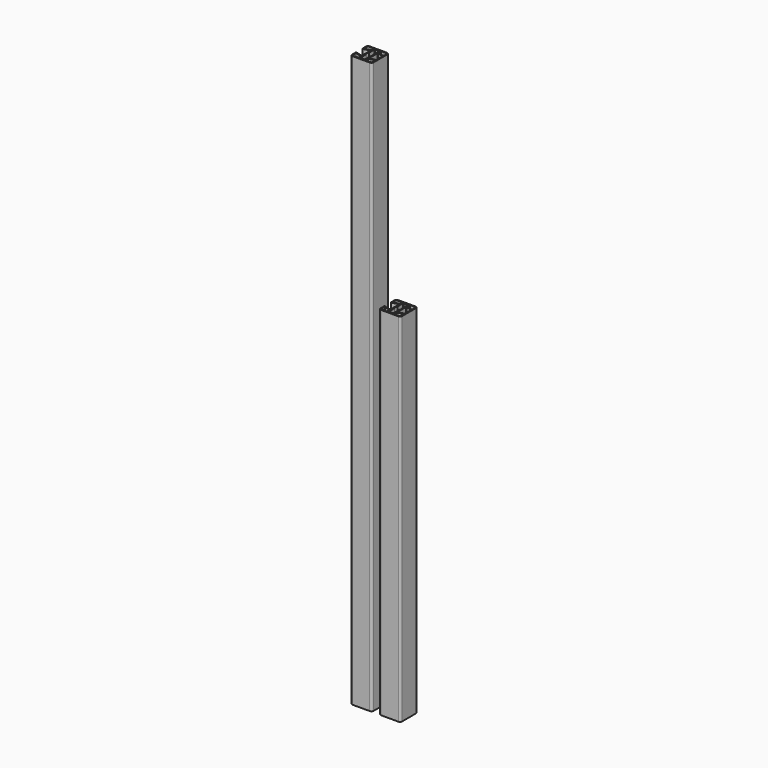
from build123d import *

# Parameters (mm, degrees)
F1_DEPTH = 1600
F2_DEPTH = 1000


# Not quite as in the source:
# - ends of sketch curves that miss each other by under 0.0002 mm in the source are joined


with BuildPart() as f1:
    # F0 (on Top) → F1 (new body)
    with BuildSketch(Plane.XY):
        with BuildLine():
            ThreePointArc((-11.2588189596, 15.2716838492), (-10.3912385359, 15.0991113133), (-10, 14.305758))
            Line((-10, 14.305758), (-10, -14.305758))
            ThreePointArc((-10, -14.305758), (-10.3912385359, -15.0991113133), (-11.2588189596, -15.2716838492))
            Line((-11.2588189596, -15.2716838492), (-28.426476, -10.671624))
            ThreePointArc((-28.426476, -10.671624), (-29.5109517857, -10.8873403242), (-30, -11.879032))
            Line((-30, -11.879032), (-30, -24))
            ThreePointArc((-30, -24), (-28.2426406871, -28.2426406871), (-24, -30))
            Line((-24, -30), (24, -30))
            ThreePointArc((24, -30), (28.2426406871, -28.2426406871), (30, -24))
            Line((30, -24), (30, 24))
            ThreePointArc((30, 24), (28.2426406871, 28.2426406871), (24, 30))
            Line((24, 30), (-24, 30))
            ThreePointArc((-24, 30), (-28.2426406871, 28.2426406871), (-30, 24))
            Line((-30, 24), (-30, 11.879032))
            ThreePointArc((-30, 11.879032), (-29.5109517857, 10.8873403242), (-28.4264761923, 10.6716247175))
            Line((-28.4264761923, 10.6716247175), (-11.2588189596, 15.2716838492))
        make_face()
        with BuildLine():
            Line((-11, -27.25), (-24, -27.25))
            ThreePointArc((-24, -27.25), (-26.2980970389, -26.2980970389), (-27.25, -24))
            Line((-27.25, -24), (-27.25, -15.137095))
            ThreePointArc((-27.25, -15.137095), (-26.8587614641, -14.3437416867), (-25.9911810404, -14.1711691508))
            Line((-25.9911810404, -14.1711691508), (-10.741181, -18.257395))
            ThreePointArc((-10.741181, -18.257395), (-10.2066466079, -18.6145586385), (-10, -19.22332))
            Line((-10, -19.22332), (-10, -26.25))
            ThreePointArc((-10, -26.25), (-10.2928932188, -26.9571067812), (-11, -27.25))
        make_face(mode=Mode.SUBTRACT)
        with BuildLine():
            Line((10.741181, -18.257395), (25.991181, -14.171169))
            ThreePointArc((25.991181, -14.171169), (26.8587614641, -14.3437416867), (27.25, -15.137095))
            Line((27.25, -15.137095), (27.25, -24))
            ThreePointArc((27.25, -24), (26.2980970389, -26.2980970389), (24, -27.25))
            Line((24, -27.25), (11, -27.25))
            ThreePointArc((11, -27.25), (10.2928932188, -26.9571067812), (10, -26.25))
            Line((10, -26.25), (10, -19.22332))
            ThreePointArc((10, -19.22332), (10.2066466079, -18.6145586385), (10.741181, -18.257395))
        make_face(mode=Mode.SUBTRACT)
        with BuildLine():
            Line((-5.2, 25.2), (5.2, 25.2))
            ThreePointArc((5.2, 25.2), (5.9071067812, 24.9071067812), (6.2, 24.2))
            Line((6.2, 24.2), (6.2, 5.4))
            ThreePointArc((6.2, 5.4), (6.2513167019, 5.083772234), (6.4, 4.8))
            ThreePointArc((6.4, 4.8), (8, 0), (6.4, -4.8))
            ThreePointArc((6.4, -4.8), (6.2513167019, -5.083772234), (6.2, -5.4))
            Line((6.2, -5.4), (6.2, -24.2))
            ThreePointArc((6.2, -24.2), (5.9071067812, -24.9071067812), (5.2, -25.2))
            Line((5.2, -25.2), (-5.2, -25.2))
            ThreePointArc((-5.2, -25.2), (-5.9071067812, -24.9071067812), (-6.2, -24.2))
            Line((-6.2, -24.2), (-6.2, -5.4))
            ThreePointArc((-6.2, -5.4), (-6.2513167019, -5.083772234), (-6.4, -4.8))
            ThreePointArc((-6.4, -4.8), (-8, 0), (-6.4, 4.8))
            ThreePointArc((-6.4, 4.8), (-6.2513167019, 5.083772234), (-6.2, 5.4))
            Line((-6.2, 5.4), (-6.2, 24.2))
            ThreePointArc((-6.2, 24.2), (-5.9071067812, 24.9071067812), (-5.2, 25.2))
        make_face(mode=Mode.SUBTRACT)
        with BuildLine():
            Line((26.87941, -11.08616), (11.258819, -15.271684))
            ThreePointArc((11.258819, -15.271684), (10.3912385359, -15.0991113133), (10, -14.305758))
            Line((10, -14.305758), (10, 14.305758))
            ThreePointArc((10, 14.305758), (10.3912385359, 15.0991113133), (11.2588189596, 15.2716838492))
            Line((11.2588189596, 15.2716838492), (26.87941, 11.08616))
            ThreePointArc((26.87941, 11.08616), (27.1466768037, 10.9075775405), (27.25, 10.603197))
            Line((27.25, 10.603197), (27.25, -10.603197))
            ThreePointArc((27.25, -10.603197), (27.1466768037, -10.9075775405), (26.87941, -11.08616))
        make_face(mode=Mode.SUBTRACT)
        with BuildLine():
            Line((-10.741181, 18.257395), (-25.991181, 14.171169))
            ThreePointArc((-25.991181, 14.171169), (-26.8587614641, 14.3437416867), (-27.25, 15.137095))
            Line((-27.25, 15.137095), (-27.25, 24))
            ThreePointArc((-27.25, 24), (-26.2980970389, 26.2980970389), (-24, 27.25))
            Line((-24, 27.25), (-11, 27.25))
            ThreePointArc((-11, 27.25), (-10.2928932188, 26.9571067812), (-10, 26.25))
            Line((-10, 26.25), (-10, 19.22332))
            ThreePointArc((-10, 19.22332), (-10.2066466079, 18.6145586385), (-10.741181, 18.257395))
        make_face(mode=Mode.SUBTRACT)
        with BuildLine():
            Line((11, 27.25), (24, 27.25))
            ThreePointArc((24, 27.25), (26.2980970389, 26.2980970389), (27.25, 24))
            Line((27.25, 24), (27.25, 15.137095))
            ThreePointArc((27.25, 15.137095), (26.8587614641, 14.3437416867), (25.9911810404, 14.1711691508))
            Line((25.9911810404, 14.1711691508), (10.741181, 18.257395))
            ThreePointArc((10.741181, 18.257395), (10.2066466079, 18.6145586385), (10, 19.22332))
            Line((10, 19.22332), (10, 26.25))
            ThreePointArc((10, 26.25), (10.2928932188, 26.9571067812), (11, 27.25))
        make_face(mode=Mode.SUBTRACT)
    extrude(amount=F1_DEPTH)


with BuildPart() as f2:
    # F0 (on Top) → F2 (new body)
    with BuildSketch(Plane.XY):
        with BuildLine():
            Line((50, -11.879032), (50, -24))
            ThreePointArc((50, -24), (51.7573593129, -28.2426406871), (56, -30))
            Line((56, -30), (104, -30))
            ThreePointArc((104, -30), (108.2426406871, -28.2426406871), (110, -24))
            Line((110, -24), (110, 24))
            ThreePointArc((110, 24), (108.2426406871, 28.2426406871), (104, 30))
            Line((104, 30), (56, 30))
            ThreePointArc((56, 30), (51.7573593129, 28.2426406871), (50, 24))
            Line((50, 24), (50, 11.879032))
            ThreePointArc((50, 11.879032), (50.4890482143, 10.8873403242), (51.5735238077, 10.6716247175))
            Line((51.5735238077, 10.6716247175), (68.741181, 15.271684))
            ThreePointArc((68.741181, 15.271684), (69.6087614641, 15.0991113133), (70, 14.305758))
            Line((70, 14.305758), (70, -14.305758))
            ThreePointArc((70, -14.305758), (69.6087614641, -15.0991113133), (68.7411810404, -15.2716838492))
            Line((68.7411810404, -15.2716838492), (51.573524, -10.671624))
            ThreePointArc((51.573524, -10.671624), (50.4890482143, -10.8873403242), (50, -11.879032))
        make_face()
        with BuildLine():
            Line((52.75, -24), (52.75, -15.137095))
            ThreePointArc((52.75, -15.137095), (53.1412385359, -14.3437416867), (54.0088189596, -14.1711691508))
            Line((54.0088189596, -14.1711691508), (69.258819, -18.257395))
            ThreePointArc((69.258819, -18.257395), (69.7933533921, -18.6145586385), (70, -19.22332))
            Line((70, -19.22332), (70, -26.25))
            ThreePointArc((70, -26.25), (69.7071067812, -26.9571067812), (69, -27.25))
            Line((69, -27.25), (56, -27.25))
            ThreePointArc((56, -27.25), (53.7019029611, -26.2980970389), (52.75, -24))
        make_face(mode=Mode.SUBTRACT)
        with BuildLine():
            ThreePointArc((107.25, -24), (106.2980970389, -26.2980970389), (104, -27.25))
            Line((104, -27.25), (91, -27.25))
            ThreePointArc((91, -27.25), (90.2928932188, -26.9571067812), (90, -26.25))
            Line((90, -26.25), (90, -19.22332))
            ThreePointArc((90, -19.22332), (90.2066466079, -18.6145586385), (90.7411807904, -18.2573942178))
            Line((90.7411807904, -18.2573942178), (105.991181, -14.171169))
            ThreePointArc((105.991181, -14.171169), (106.8587614641, -14.3437416867), (107.25, -15.137095))
            Line((107.25, -15.137095), (107.25, -24))
        make_face(mode=Mode.SUBTRACT)
        with BuildLine():
            Line((73.8, 5.4), (73.8, 24.2))
            ThreePointArc((73.8, 24.2), (74.0928932188, 24.9071067812), (74.8, 25.2))
            Line((74.8, 25.2), (85.2, 25.2))
            ThreePointArc((85.2, 25.2), (85.9071067812, 24.9071067812), (86.2, 24.2))
            Line((86.2, 24.2), (86.2, 5.4))
            ThreePointArc((86.2, 5.4), (86.2513167019, 5.083772234), (86.4, 4.8))
            ThreePointArc((86.4, 4.8), (88, 0), (86.4, -4.8))
            ThreePointArc((86.4, -4.8), (86.2513167019, -5.083772234), (86.2, -5.4))
            Line((86.2, -5.4), (86.2, -24.2))
            ThreePointArc((86.2, -24.2), (85.9071067812, -24.9071067812), (85.2, -25.2))
            Line((85.2, -25.2), (74.8, -25.2))
            ThreePointArc((74.8, -25.2), (74.0928932188, -24.9071067812), (73.8, -24.2))
            Line((73.8, -24.2), (73.8, -5.4))
            ThreePointArc((73.8, -5.4), (73.7486832981, -5.083772234), (73.6, -4.8))
            ThreePointArc((73.6, -4.8), (72, 0), (73.6, 4.8))
            ThreePointArc((73.6, 4.8), (73.7486832981, 5.083772234), (73.8, 5.4))
        make_face(mode=Mode.SUBTRACT)
        with BuildLine():
            Line((106.87941, -11.08616), (91.258819, -15.271684))
            ThreePointArc((91.258819, -15.271684), (90.3912385359, -15.0991113133), (90, -14.305758))
            Line((90, -14.305758), (90, 14.305758))
            ThreePointArc((90, 14.305758), (90.3912385359, 15.0991113133), (91.2588189596, 15.2716838492))
            Line((91.2588189596, 15.2716838492), (106.87941, 11.08616))
            ThreePointArc((106.87941, 11.08616), (107.1466768037, 10.9075775405), (107.25, 10.603197))
            Line((107.25, 10.603197), (107.25, -10.603197))
            ThreePointArc((107.25, -10.603197), (107.1466768037, -10.9075775405), (106.87941, -11.08616))
        make_face(mode=Mode.SUBTRACT)
        with BuildLine():
            ThreePointArc((52.75, 24), (53.7019029611, 26.2980970389), (56, 27.25))
            Line((56, 27.25), (69, 27.25))
            ThreePointArc((69, 27.25), (69.7071067812, 26.9571067812), (70, 26.25))
            Line((70, 26.25), (70, 19.22332))
            ThreePointArc((70, 19.22332), (69.7933533921, 18.6145586385), (69.2588192096, 18.2573942178))
            Line((69.2588192096, 18.2573942178), (54.008819, 14.171169))
            ThreePointArc((54.008819, 14.171169), (53.1412385359, 14.3437416867), (52.75, 15.137095))
            Line((52.75, 15.137095), (52.75, 24))
        make_face(mode=Mode.SUBTRACT)
        with BuildLine():
            ThreePointArc((104, 27.25), (106.2980970389, 26.2980970389), (107.25, 24))
            Line((107.25, 24), (107.25, 15.137095))
            ThreePointArc((107.25, 15.137095), (106.8587614641, 14.3437416867), (105.9911810404, 14.1711691508))
            Line((105.9911810404, 14.1711691508), (90.741181, 18.257395))
            ThreePointArc((90.741181, 18.257395), (90.2066466079, 18.6145586385), (90, 19.22332))
            Line((90, 19.22332), (90, 26.25))
            ThreePointArc((90, 26.25), (90.2928932188, 26.9571067812), (91, 27.25))
            Line((91, 27.25), (104, 27.25))
        make_face(mode=Mode.SUBTRACT)
    extrude(amount=F2_DEPTH)


solid = Compound([f1.part, f2.part])
